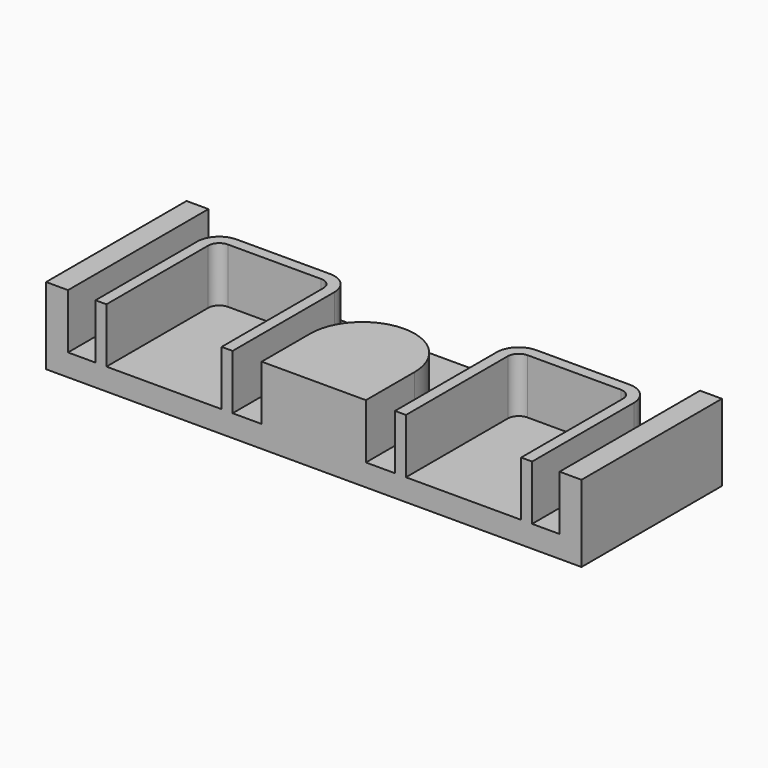
from build123d import *

# Parameters (mm, degrees)
F0_W     = 44.8
F0_H     = 16
F1_DEPTH = 2
F4_DEPTH = 5
F5_DEPTH = 5
F6_W     = 2
F6_H     = 16
F7_DEPTH = 7


# Not quite as in the source:
# - a pattern or mirror of a feature is missing from the dataset's text; its kind, count and spacing are read off the source's solid


with BuildPart() as f1:
    # F0 (on Top) → F1 (new body)
    with BuildSketch(Plane.XY):
        Rectangle(F0_W, F0_H)
    extrude(amount=F1_DEPTH)

    # F2 (on face) → F4 (join)
    with BuildSketch(Plane.XY.offset(2)):
        with BuildLine():
            Line((-19.9, 3.6), (-19.9, -8))
            Line((-19.9, -8), (-18.9, -8))
            Line((-18.9, -8), (-18.9, 3.6))
            ThreePointArc((-18.9, 3.6), (-18.6071067812, 4.3071067812), (-17.9, 4.6))
            Line((-17.9, 4.6), (-9.4, 4.6))
            ThreePointArc((-9.4, 4.6), (-8.6928932188, 4.3071067812), (-8.4, 3.6))
            Line((-8.4, 3.6), (-8.4, -8))
            Line((-8.4, -8), (-7.4, -8))
            Line((-7.4, -8), (-7.4, 3.6))
            ThreePointArc((-7.4, 3.6), (-7.9857864376, 5.0142135624), (-9.4, 5.6))
            Line((-9.4, 5.6), (-17.9, 5.6))
            ThreePointArc((-17.9, 5.6), (-19.3142135624, 5.0142135624), (-19.9, 3.6))
        make_face()
    f4 = extrude(amount=F4_DEPTH)

    # F4_copies: F4 across plane
    add(f4.mirror(Plane(origin=(0, 0, 0), x_dir=(0, 0, 1), z_dir=(1, 0, 0))))

    # F3 (on face) → F5 (join)
    with BuildSketch(Plane.XY.offset(2)):
        with BuildLine():
            Line((4.75, -8), (4.75, -2.45))
            ThreePointArc((4.75, -2.45), (0, 2.3), (-4.75, -2.45))
            Line((-4.75, -2.45), (-4.75, -8))
            Line((-4.75, -8), (4.75, -8))
        make_face()
    extrude(amount=F5_DEPTH)

    # F6 (on Top) → F7 (join, through all)
    with BuildSketch(Plane.XY):
        with Locations((-23.4, 0)):
            Rectangle(F6_W, F6_H)
    f7 = extrude(amount=F7_DEPTH)

    # F7_copies: F7 across plane
    add(f7.mirror(Plane(origin=(0, 0, 0), x_dir=(0, 0, 1), z_dir=(1, 0, 0))))


solid = f1.part
